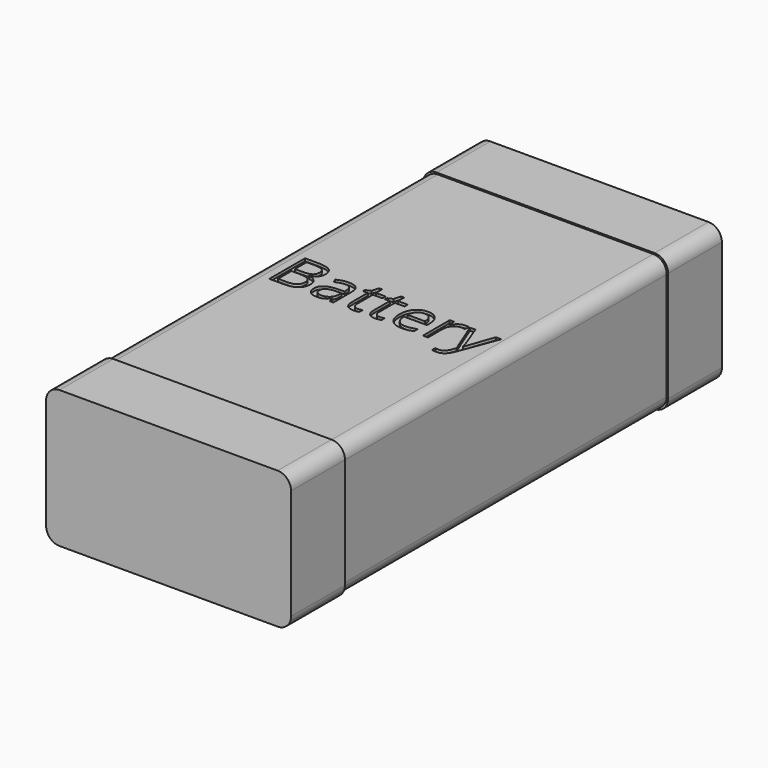
from build123d import *

# Parameters (mm, degrees)
F0_W         = 90
F0_H         = 50
F1_DEPTH     = 200
F2_TEXT_SIZE = 23.2073248119
F3_DEPTH     = 1
F4_W         = 91
F4_H         = 51
F4_W_2       = 90
F4_H_2       = 50
F5_DEPTH     = 25
F6_W         = 91
F6_H         = 51
F6_W_2       = 90
F6_H_2       = 50
F7_DEPTH     = 25
F8_R         = 5


# Not quite as in the source:
# - Text() gives the source's letters only with a copy of the font that has no kerning and outlines rounded to 1/6400 em; it was checked with that copy


with BuildPart() as f1:
    # F0 (on Front) → F1 (new body)
    with BuildSketch(Plane.XZ):
        with Locations((45, 25)):
            Rectangle(F0_W, F0_H)
    extrude(amount=F1_DEPTH)

    # F2 (on face) → F3 (cut)
    with BuildSketch(Plane.XY.offset(50)):
        with Locations((5.5, -106.7092738646)):
            Text('Battery', F2_TEXT_SIZE, font='Open Sans', text_align=(TextAlign.LEFT, TextAlign.BOTTOM))
    extrude(amount=-F3_DEPTH, mode=Mode.SUBTRACT)

    # F4 (on face) → F5 (join)
    with BuildSketch(Plane.XZ.offset(200)):
        with Locations((45, 25)):
            Rectangle(F4_W, F4_H)
        with Locations((45, 25)):
            Rectangle(F4_W_2, F4_H_2, mode=Mode.SUBTRACT)
    extrude(amount=-F5_DEPTH)

    # F6 (on face) → F7 (join)
    with BuildSketch(Plane(origin=(0, 0, 0), x_dir=(-1, 0, 0), z_dir=(0, 1, 0))):
        with Locations((-45, 25)):
            Rectangle(F6_W, F6_H)
        with Locations((-45, 25)):
            Rectangle(F6_W_2, F6_H_2, mode=Mode.SUBTRACT)
    extrude(amount=-F7_DEPTH)

    # F8
    f8_edges = [f1.edges().sort_by_distance(p)[0] for p in [
        (90, -100, 50),
        (0, -100, 50),
        (90, -100, 0),
        (0, -100, 0),
        (90.5, -12.5, 50.5),
        (-0.5, -12.5, 50.5),
        (90.5, -12.5, -0.5),
        (-0.5, -12.5, -0.5),
        (-0.5, -187.5, 50.5),
        (-0.5, -187.5, -0.5),
        (90.5, -187.5, 50.5),
        (90.5, -187.5, -0.5),
    ]]
    fillet(f8_edges, radius=F8_R)


solid = f1.part
